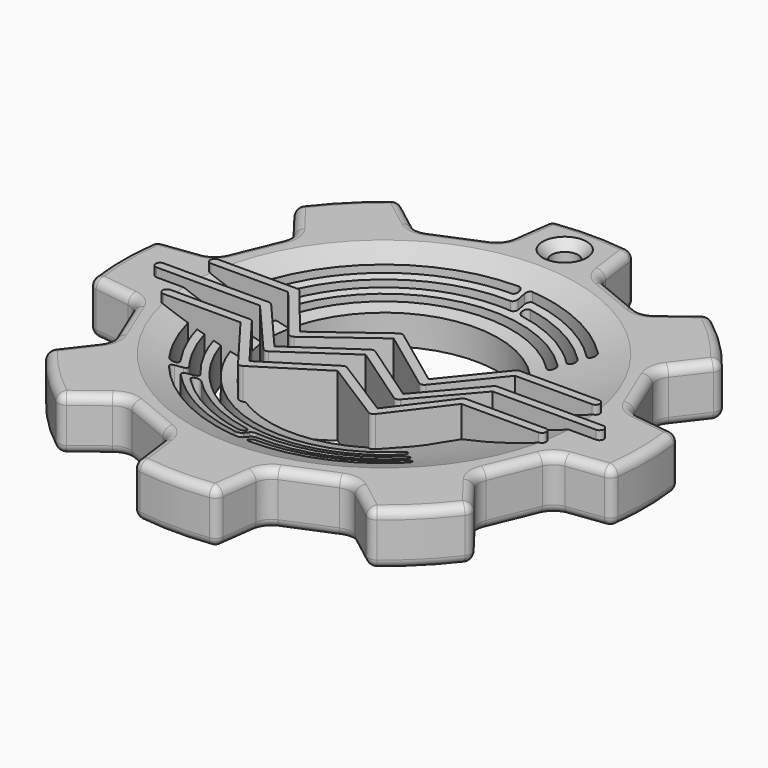
from build123d import *

# Parameters (mm, degrees)
F1_R          = 65
F3_DEPTH      = 15
F4_ANGLE      = 22.5
F5_DEPTH      = 37
F6_R          = 2.5
F7_R          = 10
F9_ANGLE_BACK = 42.021197958
F9_ANGLE      = 84.0423959161
F11_DEPTH     = 20
F12_DEPTH     = 15
F13_R         = 5
F14_R         = 7.5
F15_DEPTH     = 30.0010001
F16_SIZE      = 5


with BuildPart() as f3:
    # F1 (on Top) → F3 (new body, symmetric)
    with BuildSketch(Plane.XY):
        with BuildLine():
            Line((119.8787593446, 20), (145.8595214581, 35))
            ThreePointArc((145.8595214581, 35), (138.5819298767, 57.4025148548), (127.8869940652, 78.3895193822))
            Line((127.8869940652, 78.3895193822), (98.9092192765, 70.6249480291))
            Line((98.9092192765, 70.6249480291), (70.6249480291, 98.9092192765))
            Line((70.6249480291, 98.9092192765), (78.3895193822, 127.8869940652))
            ThreePointArc((78.3895193822, 127.8869940652), (57.4025148548, 138.5819298767), (35, 145.8595214581))
            Line((35, 145.8595214581), (20, 119.8787593446))
            Line((20, 119.8787593446), (-20, 119.8787593446))
            Line((-20, 119.8787593446), (-35, 145.8595214581))
            ThreePointArc((-35, 145.8595214581), (-57.4025148548, 138.5819298767), (-78.3895193822, 127.8869940652))
            Line((-78.3895193822, 127.8869940652), (-70.6249480291, 98.9092192765))
            Line((-70.6249480291, 98.9092192765), (-98.9092192765, 70.6249480291))
            Line((-98.9092192765, 70.6249480291), (-127.8869940652, 78.3895193822))
            ThreePointArc((-127.8869940652, 78.3895193822), (-138.5819298767, 57.4025148548), (-145.8595214581, 35))
            Line((-145.8595214581, 35), (-119.8787593446, 20))
            Line((-119.8787593446, 20), (-119.8787593446, -20))
            Line((-119.8787593446, -20), (-145.8595214581, -35))
            ThreePointArc((-145.8595214581, -35), (-138.5819298767, -57.4025148548), (-127.8869940652, -78.3895193822))
            Line((-127.8869940652, -78.3895193822), (-98.9092192765, -70.6249480291))
            Line((-98.9092192765, -70.6249480291), (-70.6249480291, -98.9092192765))
            Line((-70.6249480291, -98.9092192765), (-78.3895193822, -127.8869940652))
            ThreePointArc((-78.3895193822, -127.8869940652), (-57.4025148548, -138.5819298767), (-35, -145.8595214581))
            Line((-35, -145.8595214581), (-20, -119.8787593446))
            Line((-20, -119.8787593446), (20, -119.8787593446))
            Line((20, -119.8787593446), (35, -145.8595214581))
            ThreePointArc((35, -145.8595214581), (57.4025148548, -138.5819298767), (78.3895193822, -127.8869940652))
            Line((78.3895193822, -127.8869940652), (70.6249480291, -98.9092192765))
            Line((70.6249480291, -98.9092192765), (98.9092192765, -70.6249480291))
            Line((98.9092192765, -70.6249480291), (127.8869940652, -78.3895193822))
            ThreePointArc((127.8869940652, -78.3895193822), (138.5819298767, -57.4025148548), (145.8595214581, -35))
            Line((145.8595214581, -35), (119.8787593446, -20))
            Line((119.8787593446, -20), (119.8787593446, 20))
        make_face()
        Circle(F1_R, mode=Mode.SUBTRACT)
    extrude(amount=F3_DEPTH, both=True)


with BuildPart() as f3_1:
    # F4: moved
    add(f3.part.rotate(Axis((0, 0, -15), (0, 0, 1)), F4_ANGLE))

    # F0 (on Top) → F5 (cut, symmetric)
    with BuildSketch(Plane.XY):
        with BuildLine():
            ThreePointArc((51.265241636, 51.265241636), (54.800775542, 51.265241636), (54.800775542, 54.800775542))
            ThreePointArc((54.800775542, 54.800775542), (-77.5, 0), (54.800775542, -54.800775542))
            ThreePointArc((54.800775542, -54.800775542), (54.800775542, -51.265241636), (51.265241636, -51.265241636))
            ThreePointArc((51.265241636, -51.265241636), (-72.5, 0), (51.265241636, 51.265241636))
        make_face()
        with BuildLine():
            ThreePointArc((57.6292026667, 57.6292026667), (61.1647365726, 57.6292026667), (61.1647365726, 61.1647365726))
            ThreePointArc((61.1647365726, 61.1647365726), (39.9412550448, 76.7264370699), (15.0205673682, 85.1858706356))
            ThreePointArc((15.0205673682, 85.1858706356), (12.1244275415, 83.1579716972), (14.1523264799, 80.2618318705))
            ThreePointArc((14.1523264799, 80.2618318705), (37.6325119787, 72.291382904), (57.6292026667, 57.6292026667))
        make_face()
        with BuildLine():
            ThreePointArc((-62.7407641978, -55.9092703215), (-64.5656225789, -56.4846459589), (-66.2628443298, -55.6011282379))
            Line((-66.2628443298, -55.6011282379), (-69.3270221023, -58.1722786766))
            ThreePointArc((-69.3270221023, -58.1722786766), (-68.5168463916, -59.1243753502), (-67.6935962189, -60.0651898437))
            Line((-67.6935962189, -60.0651898437), (-62.7407641978, -55.9092703215))
        make_face()
        with BuildLine():
            ThreePointArc((-67.8421325563, -53.6627901829), (-67.0594922066, -54.6376656254), (-66.2628443298, -55.6011282379))
            ThreePointArc((-66.2628443298, -55.6011282379), (-64.5656225789, -56.4846459589), (-62.7407641978, -55.9092703215))
            ThreePointArc((-62.7407641978, -55.9092703215), (-61.8572464768, -54.2120485705), (-62.4326221142, -52.3871901895))
            ThreePointArc((-62.4326221142, -52.3871901895), (-64.1298438651, -51.5036724684), (-65.9547022462, -52.0790481059))
            Line((-65.9547022462, -52.0790481059), (-67.8421325563, -53.6627901829))
        make_face()
        with BuildLine():
            Line((-69.3270221023, -58.1722786766), (-66.2628443298, -55.6011282379))
            ThreePointArc((-66.2628443298, -55.6011282379), (-67.0594922066, -54.6376656254), (-67.8421325563, -53.6627901829))
            Line((-67.8421325563, -53.6627901829), (-72.8491022343, -57.8641365931))
            ThreePointArc((-72.8491022343, -57.8641365931), (-71.0242438532, -57.2887609556), (-69.3270221023, -58.1722786766))
        make_face()
        with BuildLine():
            ThreePointArc((-67.6935962189, -60.0651898437), (-68.5168463916, -59.1243753502), (-69.3270221023, -58.1722786766))
            ThreePointArc((-69.3270221023, -58.1722786766), (-71.0242438532, -57.2887609556), (-72.8491022343, -57.8641365931))
            ThreePointArc((-72.8491022343, -57.8641365931), (-73.7326199553, -59.561358344), (-73.1572443179, -61.3862167251))
            ThreePointArc((-73.1572443179, -61.3862167251), (-71.4600225669, -62.2697344461), (-69.6351641858, -61.6943588086))
            Line((-69.6351641858, -61.6943588086), (-67.6935962189, -60.0651898437))
        make_face()
        with BuildLine():
            ThreePointArc((5.0453356545, 86.3527335302), (-76.7264370699, 39.9412550448), (-67.8421325563, -53.6627901829))
            Line((-67.8421325563, -53.6627901829), (-65.9547022462, -52.0790481059))
            ThreePointArc((-65.9547022462, -52.0790481059), (-64.1298438651, -51.5036724684), (-62.4326221142, -52.3871901895))
            ThreePointArc((-62.4326221142, -52.3871901895), (-72.291382904, 37.6325119787), (7.1031930339, 81.1898678945))
            ThreePointArc((7.1031930339, 81.1898678945), (5.405971283, 82.0733856155), (4.8305956456, 83.8982439966))
            Line((4.8305956456, 83.8982439966), (5.0453356545, 86.3527335302))
        make_face()
        with BuildLine():
            ThreePointArc((-10.375071368, -89.9033252672), (-41.7882494978, -80.2744804026), (-67.6935962189, -60.0651898437))
            Line((-67.6935962189, -60.0651898437), (-69.6351641858, -61.6943588086))
            ThreePointArc((-69.6351641858, -61.6943588086), (-71.4600225669, -62.2697344461), (-73.1572443179, -61.3862167251))
            ThreePointArc((-73.1572443179, -61.3862167251), (-44.0969925639, -84.7095345685), (-8.3233734324, -95.1365936678))
            ThreePointArc((-8.3233734324, -95.1365936678), (-10.0205951833, -94.2530759467), (-10.5959708208, -92.4282175657))
            Line((-10.5959708208, -92.4282175657), (-10.375071368, -89.9033252672))
        make_face()
        with BuildLine():
            ThreePointArc((7.5389717477, 86.1708413849), (6.2928109289, 86.27079767), (5.0453356545, 86.3527335302))
            Line((5.0453356545, 86.3527335302), (4.8305956456, 83.8982439966))
            ThreePointArc((4.8305956456, 83.8982439966), (5.405971283, 82.0733856155), (7.1031930339, 81.1898678945))
            ThreePointArc((7.1031930339, 81.1898678945), (8.928051415, 81.7652435319), (9.811569136, 83.4624652828))
            ThreePointArc((9.811569136, 83.4624652828), (9.2361934986, 85.2873236639), (7.5389717477, 86.1708413849))
        make_face()
        with BuildLine():
            Line((5.6149973303, 92.8639962794), (5.0453356545, 86.3527335302))
            ThreePointArc((5.0453356545, 86.3527335302), (6.2928109289, 86.27079767), (7.5389717477, 86.1708413849))
            ThreePointArc((7.5389717477, 86.1708413849), (9.2361934986, 85.2873236639), (9.811569136, 83.4624652828))
            Line((9.811569136, 83.4624652828), (10.375071368, 89.9033252672))
            ThreePointArc((10.375071368, 89.9033252672), (9.1322043521, 90.0380633048), (7.8875947187, 90.1556201773))
            ThreePointArc((7.8875947187, 90.1556201773), (6.1903729677, 91.0391378983), (5.6149973303, 92.8639962794))
        make_face()
        with BuildLine():
            ThreePointArc((-7.8875947187, -90.1556201773), (-9.1322043521, -90.0380633048), (-10.375071368, -89.9033252672))
            Line((-10.375071368, -89.9033252672), (-10.5959708208, -92.4282175657))
            ThreePointArc((-10.5959708208, -92.4282175657), (-10.0205951833, -94.2530759467), (-8.3233734324, -95.1365936678))
            ThreePointArc((-8.3233734324, -95.1365936678), (-6.4985150513, -94.5612180303), (-5.6149973303, -92.8639962794))
            ThreePointArc((-5.6149973303, -92.8639962794), (-6.1903729677, -91.0391378983), (-7.8875947187, -90.1556201773))
        make_face()
        with BuildLine():
            Line((-9.811569136, -83.4624652828), (-10.375071368, -89.9033252672))
            ThreePointArc((-10.375071368, -89.9033252672), (-9.1322043521, -90.0380633048), (-7.8875947187, -90.1556201773))
            ThreePointArc((-7.8875947187, -90.1556201773), (-6.1903729677, -91.0391378983), (-5.6149973303, -92.8639962794))
            Line((-5.6149973303, -92.8639962794), (-5.0453356545, -86.3527335302))
            ThreePointArc((-5.0453356545, -86.3527335302), (-6.2928109289, -86.27079767), (-7.5389717477, -86.1708413849))
            ThreePointArc((-7.5389717477, -86.1708413849), (-9.2361934986, -85.2873236639), (-9.811569136, -83.4624652828))
        make_face()
        with BuildLine():
            ThreePointArc((8.3233734324, 95.1365936678), (6.4985150513, 94.5612180303), (5.6149973303, 92.8639962794))
            ThreePointArc((5.6149973303, 92.8639962794), (6.1903729677, 91.0391378983), (7.8875947187, 90.1556201773))
            ThreePointArc((7.8875947187, 90.1556201773), (9.1322043521, 90.0380633048), (10.375071368, 89.9033252672))
            Line((10.375071368, 89.9033252672), (10.5959708208, 92.4282175657))
            ThreePointArc((10.5959708208, 92.4282175657), (10.0205951833, 94.2530759467), (8.3233734324, 95.1365936678))
        make_face()
        with BuildLine():
            ThreePointArc((-7.1031930339, -81.1898678945), (-8.928051415, -81.7652435319), (-9.811569136, -83.4624652828))
            ThreePointArc((-9.811569136, -83.4624652828), (-9.2361934986, -85.2873236639), (-7.5389717477, -86.1708413849))
            ThreePointArc((-7.5389717477, -86.1708413849), (-6.2928109289, -86.27079767), (-5.0453356545, -86.3527335302))
            Line((-5.0453356545, -86.3527335302), (-4.8305956456, -83.8982439966))
            ThreePointArc((-4.8305956456, -83.8982439966), (-5.405971283, -82.0733856155), (-7.1031930339, -81.1898678945))
        make_face()
        with BuildLine():
            ThreePointArc((67.5286976033, 67.5286976033), (40.3600439962, 86.552393662), (8.3233734324, 95.1365936678))
            ThreePointArc((8.3233734324, 95.1365936678), (10.0205951833, 94.2530759467), (10.5959708208, 92.4282175657))
            Line((10.5959708208, 92.4282175657), (10.375071368, 89.9033252672))
            ThreePointArc((10.375071368, 89.9033252672), (39.3762963575, 81.4847058359), (63.9931636974, 63.9931636974))
            ThreePointArc((63.9931636974, 63.9931636974), (67.5286976033, 63.9931636974), (67.5286976033, 67.5286976033))
        make_face()
        with BuildLine():
            ThreePointArc((57.6292026667, -57.6292026667), (27.874641681, -76.5849485941), (-7.1031930339, -81.1898678945))
            ThreePointArc((-7.1031930339, -81.1898678945), (-5.405971283, -82.0733856155), (-4.8305956456, -83.8982439966))
            Line((-4.8305956456, -83.8982439966), (-5.0453356545, -86.3527335302))
            ThreePointArc((-5.0453356545, -86.3527335302), (30.7563910031, -80.8473525384), (61.1647365726, -61.1647365726))
            ThreePointArc((61.1647365726, -61.1647365726), (61.1647365726, -57.6292026667), (57.6292026667, -57.6292026667))
        make_face()
        with BuildLine():
            ThreePointArc((0, 90.5), (2.5, 93), (0, 95.5))
            ThreePointArc((0, 95.5), (-84.7095345685, 44.0969925639), (-78.2290202296, -54.7765496715))
            ThreePointArc((-78.2290202296, -54.7765496715), (-74.747199028, -55.3904886914), (-74.1332600082, -51.9086674898))
            ThreePointArc((-74.1332600082, -51.9086674898), (-80.2744804026, 41.7882494978), (0, 90.5))
        make_face()
        with BuildLine():
            ThreePointArc((0, -90.5), (-2.5, -93), (0, -95.5))
            ThreePointArc((0, -95.5), (36.5462677909, -88.2304953548), (67.5286976033, -67.5286976033))
            ThreePointArc((67.5286976033, -67.5286976033), (67.5286976033, -63.9931636974), (63.9931636974, -63.9931636974))
            ThreePointArc((63.9931636974, -63.9931636974), (34.632850629, -83.6110976923), (0, -90.5))
        make_face()
        with BuildLine():
            ThreePointArc((-57.6292026667, -57.6292026667), (-61.1647365726, -57.6292026667), (-61.1647365726, -61.1647365726))
            ThreePointArc((-61.1647365726, -61.1647365726), (-39.9412550448, -76.7264370699), (-15.0205673682, -85.1858706356))
            ThreePointArc((-15.0205673682, -85.1858706356), (-12.1244275415, -83.1579716972), (-14.1523264799, -80.2618318705))
            ThreePointArc((-14.1523264799, -80.2618318705), (-37.6325119787, -72.291382904), (-57.6292026667, -57.6292026667))
        make_face()
    extrude(amount=F5_DEPTH, both=True, mode=Mode.SUBTRACT)

    # F6
    f6_edges = [f3_1.edges().sort_by_distance(p)[0] for p in [
        (-67.842133, -53.66279, 0),
        (-10.375071, -89.903325, 0),
        (-5.045336, -86.352734, 0),
        (-67.693596, -60.06519, 0),
        (10.375071, 89.903325, 0),
        (5.045336, 86.352734, 0),
    ]]
    fillet(f6_edges, radius=F6_R)

    # F7
    f7_edges = [f3_1.edges().sort_by_distance(p)[0] for p in [
        (-118.407201, 27.398024, 0),
        (-103.099863, 64.353206, 0),
        (-64.353206, 103.099863, 0),
        (-27.398024, 118.407201, 0),
        (27.398024, 118.407201, 0),
        (64.353206, 103.099863, 0),
        (103.099863, 64.353206, 0),
        (118.407201, 27.398024, 0),
        (118.407201, -27.398024, 0),
        (103.099863, -64.353206, 0),
        (64.353206, -103.099863, 0),
        (27.398024, -118.407201, 0),
        (-27.398024, -118.407201, 0),
        (-64.353206, -103.099863, 0),
        (-103.099863, -64.353206, 0),
        (-118.407201, -27.398024, 0),
    ]]
    fillet(f7_edges, radius=F7_R)


with BuildPart() as f9:
    # F8 (on Front) → F9 (revolve)
    with BuildSketch(Plane.XZ, mode=Mode.PRIVATE) as f9_sk:
        with BuildLine():
            Line((0, 305), (-310, 305))
            ThreePointArc((-310, 305), (0, -5), (310, 305))
            Line((310, 305), (0, 305))
        make_face()
    revolve(f9_sk.sketch.rotate(Axis((0, 0, 305), (1, 0, 0)), -F9_ANGLE_BACK), axis=Axis((0, 0, 305), (1, 0, 0)), revolution_arc=F9_ANGLE)


with BuildPart() as f3_2:
    add(f3_1.part)

    # F10: cut F9
    add(f9.part, mode=Mode.SUBTRACT)

    # F2 (on Top) → F11 (join)
    with BuildSketch(Plane.XY):
        with BuildLine():
            ThreePointArc((-106.5142259969, -18.5), (-109.0142259969, -21), (-106.5142259969, -23.5))
            Line((-106.5142259969, -23.5), (-62.7586036079, -23.5))
            Line((-62.7586036079, -23.5), (-63.5088106899, -22.5071933859))
            ThreePointArc((-63.5088106899, -22.5071933859), (-63.7523036838, -19.8859944939), (-61.5142259969, -18.5))
            Line((-61.5142259969, -18.5), (-106.5142259969, -18.5))
        make_face()
        with BuildLine():
            Line((-63.5088106899, -22.5071933859), (-62.7586036079, -23.5))
            Line((-62.7586036079, -23.5), (-61.5142259969, -23.5))
            ThreePointArc((-61.5142259969, -23.5), (-59.2761483101, -22.1140055061), (-59.5196413039, -19.4928066141))
            ThreePointArc((-59.5196413039, -19.4928066141), (-60.4002204908, -18.7619223131), (-61.5142259969, -18.5))
            ThreePointArc((-61.5142259969, -18.5), (-63.7523036838, -19.8859944939), (-63.5088106899, -22.5071933859))
        make_face()
        with BuildLine():
            Line((-61.5142259969, -23.5), (-62.7586036079, -23.5))
            Line((-62.7586036079, -23.5), (-38.994584693, -54.9487502495))
            ThreePointArc((-38.994584693, -54.9487502495), (-39.459840378, -52.9952550434), (-38.3379651856, -51.3297213675))
            Line((-38.3379651856, -51.3297213675), (-36.3933006484, -50.0976682776))
            Line((-36.3933006484, -50.0976682776), (-59.5196413039, -19.4928066141))
            ThreePointArc((-59.5196413039, -19.4928066141), (-59.2761483101, -22.1140055061), (-61.5142259969, -23.5))
        make_face()
        with BuildLine():
            ThreePointArc((-38.3379651856, -51.3297213675), (-39.459840378, -52.9952550434), (-38.994584693, -54.9487502495))
            ThreePointArc((-38.994584693, -54.9487502495), (-37.4463018202, -55.9013972416), (-35.6620348144, -55.5533923596))
            ThreePointArc((-35.6620348144, -55.5533923596), (-34.540159622, -53.8878586837), (-35.005415307, -51.9343634776))
            Line((-35.005415307, -51.9343634776), (-36.3933006484, -50.0976682776))
            Line((-36.3933006484, -50.0976682776), (-38.3379651856, -51.3297213675))
        make_face()
        with BuildLine():
            ThreePointArc((-35.005415307, -51.9343634776), (-34.540159622, -53.8878586837), (-35.6620348144, -55.5533923596))
            Line((-35.6620348144, -55.5533923596), (0, -32.9595108198))
            Line((0, -32.9595108198), (-1.3379651856, -32.111835496))
            ThreePointArc((-1.3379651856, -32.111835496), (-2.5, -30), (-1.3379651856, -27.888164504))
            Line((-1.3379651856, -27.888164504), (-36.3933006484, -50.0976682776))
            Line((-36.3933006484, -50.0976682776), (-35.005415307, -51.9343634776))
        make_face()
        with BuildLine():
            Line((-1.3379651856, -32.111835496), (0, -32.9595108198))
            Line((0, -32.9595108198), (1.3379651856, -32.111835496))
            ThreePointArc((1.3379651856, -32.111835496), (2.5, -30), (1.3379651856, -27.888164504))
            ThreePointArc((1.3379651856, -27.888164504), (0, -27.5), (-1.3379651856, -27.888164504))
            ThreePointArc((-1.3379651856, -27.888164504), (-2.5, -30), (-1.3379651856, -32.111835496))
        make_face()
        with BuildLine():
            Line((1.3379651856, -32.111835496), (0, -32.9595108198))
            Line((0, -32.9595108198), (35.6620348144, -55.5533923596))
            ThreePointArc((35.6620348144, -55.5533923596), (34.540159622, -53.8878586837), (35.005415307, -51.9343634776))
            Line((35.005415307, -51.9343634776), (36.3933006484, -50.0976682776))
            Line((36.3933006484, -50.0976682776), (1.3379651856, -27.888164504))
            ThreePointArc((1.3379651856, -27.888164504), (2.5, -30), (1.3379651856, -32.111835496))
        make_face()
        with BuildLine():
            ThreePointArc((35.005415307, -51.9343634776), (34.540159622, -53.8878586837), (35.6620348144, -55.5533923596))
            ThreePointArc((35.6620348144, -55.5533923596), (37.4463018202, -55.9013972416), (38.994584693, -54.9487502495))
            ThreePointArc((38.994584693, -54.9487502495), (39.459840378, -52.9952550434), (38.3379651856, -51.3297213675))
            Line((38.3379651856, -51.3297213675), (36.3933006484, -50.0976682776))
            Line((36.3933006484, -50.0976682776), (35.005415307, -51.9343634776))
        make_face()
        with BuildLine():
            ThreePointArc((38.3379651856, -51.3297213675), (39.459840378, -52.9952550434), (38.994584693, -54.9487502495))
            Line((38.994584693, -54.9487502495), (62.7586036079, -23.5))
            Line((62.7586036079, -23.5), (61.5142259969, -23.5))
            ThreePointArc((61.5142259969, -23.5), (59.2761483101, -22.1140055061), (59.5196413039, -19.4928066141))
            Line((59.5196413039, -19.4928066141), (36.3933006484, -50.0976682776))
            Line((36.3933006484, -50.0976682776), (38.3379651856, -51.3297213675))
        make_face()
        with BuildLine():
            Line((61.5142259969, -23.5), (62.7586036079, -23.5))
            Line((62.7586036079, -23.5), (63.5088106899, -22.5071933859))
            ThreePointArc((63.5088106899, -22.5071933859), (63.7523036838, -19.8859944939), (61.5142259969, -18.5))
            ThreePointArc((61.5142259969, -18.5), (60.4002204908, -18.7619223131), (59.5196413039, -19.4928066141))
            ThreePointArc((59.5196413039, -19.4928066141), (59.2761483101, -22.1140055061), (61.5142259969, -23.5))
        make_face()
        with BuildLine():
            Line((63.5088106899, -22.5071933859), (62.7586036079, -23.5))
            Line((62.7586036079, -23.5), (106.5142259969, -23.5))
            ThreePointArc((106.5142259969, -23.5), (109.0142259969, -21), (106.5142259969, -18.5))
            Line((106.5142259969, -18.5), (61.5142259969, -18.5))
            ThreePointArc((61.5142259969, -18.5), (63.7523036838, -19.8859944939), (63.5088106899, -22.5071933859))
        make_face()
        with BuildLine():
            ThreePointArc((-124.930732323, -0.5), (-127.430732323, -3), (-124.930732323, -5.5))
            Line((-124.930732323, -5.5), (-66.0772491679, -5.5))
            Line((-66.0772491679, -5.5), (-66.825300226, -4.6311383942))
            ThreePointArc((-66.825300226, -4.6311383942), (-67.2031589979, -1.9578498154), (-64.930732323, -0.5))
            Line((-64.930732323, -0.5), (-124.930732323, -0.5))
        make_face()
        with BuildLine():
            Line((-66.825300226, -4.6311383942), (-66.0772491679, -5.5))
            Line((-66.0772491679, -5.5), (-64.930732323, -5.5))
            ThreePointArc((-64.930732323, -5.5), (-62.6583056481, -4.0421501846), (-63.03616442, -1.3688616058))
            ThreePointArc((-63.03616442, -1.3688616058), (-63.8885821384, -0.7275733251), (-64.930732323, -0.5))
            ThreePointArc((-64.930732323, -0.5), (-67.2031589979, -1.9578498154), (-66.825300226, -4.6311383942))
        make_face()
        with BuildLine():
            Line((-64.930732323, -5.5), (-66.0772491679, -5.5))
            Line((-66.0772491679, -5.5), (-38.894567903, -37.0726952577))
            ThreePointArc((-38.894567903, -37.0726952577), (-39.479289508, -35.1204283293), (-38.4164754282, -33.381557504))
            Line((-38.4164754282, -33.381557504), (-36.5686042305, -32.1109434459))
            Line((-36.5686042305, -32.1109434459), (-63.03616442, -1.3688616058))
            ThreePointArc((-63.03616442, -1.3688616058), (-62.6583056481, -4.0421501846), (-64.930732323, -5.5))
        make_face()
        with BuildLine():
            ThreePointArc((-38.4164754282, -33.381557504), (-39.479289508, -35.1204283293), (-38.894567903, -37.0726952577))
            ThreePointArc((-38.894567903, -37.0726952577), (-37.3211285343, -37.9208463716), (-35.5835245718, -37.5015562231))
            ThreePointArc((-35.5835245718, -37.5015562231), (-34.520710492, -35.7626853978), (-35.105432097, -33.8104184694))
            Line((-35.105432097, -33.8104184694), (-36.5686042305, -32.1109434459))
            Line((-36.5686042305, -32.1109434459), (-38.4164754282, -33.381557504))
        make_face()
        with BuildLine():
            ThreePointArc((-35.105432097, -33.8104184694), (-34.520710492, -35.7626853978), (-35.5835245718, -37.5015562231))
            Line((-35.5835245718, -37.5015562231), (0, -13.0339815258))
            Line((0, -13.0339815258), (-1.4164754282, -12.0599993595))
            ThreePointArc((-1.4164754282, -12.0599993595), (-2.5, -10), (-1.4164754282, -7.9400006405))
            Line((-1.4164754282, -7.9400006405), (-36.5686042305, -32.1109434459))
            Line((-36.5686042305, -32.1109434459), (-35.105432097, -33.8104184694))
        make_face()
        with BuildLine():
            Line((-1.4164754282, -12.0599993595), (0, -13.0339815258))
            Line((0, -13.0339815258), (1.4164754282, -12.0599993595))
            ThreePointArc((1.4164754282, -12.0599993595), (2.5, -10), (1.4164754282, -7.9400006405))
            ThreePointArc((1.4164754282, -7.9400006405), (0, -7.5), (-1.4164754282, -7.9400006405))
            ThreePointArc((-1.4164754282, -7.9400006405), (-2.5, -10), (-1.4164754282, -12.0599993595))
        make_face()
        with BuildLine():
            Line((1.4164754282, -12.0599993595), (0, -13.0339815258))
            Line((0, -13.0339815258), (35.5835245718, -37.5015562231))
            ThreePointArc((35.5835245718, -37.5015562231), (34.520710492, -35.7626853978), (35.105432097, -33.8104184694))
            Line((35.105432097, -33.8104184694), (36.5686042305, -32.1109434459))
            Line((36.5686042305, -32.1109434459), (1.4164754282, -7.9400006405))
            ThreePointArc((1.4164754282, -7.9400006405), (2.5, -10), (1.4164754282, -12.0599993595))
        make_face()
        with BuildLine():
            ThreePointArc((35.105432097, -33.8104184694), (34.520710492, -35.7626853978), (35.5835245718, -37.5015562231))
            ThreePointArc((35.5835245718, -37.5015562231), (37.3211285343, -37.9208463716), (38.894567903, -37.0726952577))
            ThreePointArc((38.894567903, -37.0726952577), (39.479289508, -35.1204283293), (38.4164754282, -33.381557504))
            Line((38.4164754282, -33.381557504), (36.5686042305, -32.1109434459))
            Line((36.5686042305, -32.1109434459), (35.105432097, -33.8104184694))
        make_face()
        with BuildLine():
            ThreePointArc((38.4164754282, -33.381557504), (39.479289508, -35.1204283293), (38.894567903, -37.0726952577))
            Line((38.894567903, -37.0726952577), (66.0772491679, -5.5))
            Line((66.0772491679, -5.5), (64.930732323, -5.5))
            ThreePointArc((64.930732323, -5.5), (62.6583056481, -4.0421501846), (63.03616442, -1.3688616058))
            Line((63.03616442, -1.3688616058), (36.5686042305, -32.1109434459))
            Line((36.5686042305, -32.1109434459), (38.4164754282, -33.381557504))
        make_face()
        with BuildLine():
            Line((64.930732323, -5.5), (66.0772491679, -5.5))
            Line((66.0772491679, -5.5), (66.825300226, -4.6311383942))
            ThreePointArc((66.825300226, -4.6311383942), (67.2031589979, -1.9578498154), (64.930732323, -0.5))
            ThreePointArc((64.930732323, -0.5), (63.8885821384, -0.7275733251), (63.03616442, -1.3688616058))
            ThreePointArc((63.03616442, -1.3688616058), (62.6583056481, -4.0421501846), (64.930732323, -5.5))
        make_face()
        with BuildLine():
            Line((66.825300226, -4.6311383942), (66.0772491679, -5.5))
            Line((66.0772491679, -5.5), (124.930732323, -5.5))
            ThreePointArc((124.930732323, -5.5), (127.430732323, -3), (124.930732323, -0.5))
            Line((124.930732323, -0.5), (64.930732323, -0.5))
            ThreePointArc((64.930732323, -0.5), (67.2031589979, -1.9578498154), (66.825300226, -4.6311383942))
        make_face()
        with BuildLine():
            ThreePointArc((-108.2455532034, 17.5), (-110.7455532034, 15), (-108.2455532034, 12.5))
            Line((-108.2455532034, 12.5), (-64.4387094171, 12.5))
            Line((-64.4387094171, 12.5), (-65.1891533907, 13.4276074562))
            ThreePointArc((-65.1891533907, 13.4276074562), (-65.5017647803, 16.076805145), (-63.2455532034, 17.5))
            Line((-63.2455532034, 17.5), (-108.2455532034, 17.5))
        make_face()
        with BuildLine():
            Line((-65.1891533907, 13.4276074562), (-64.4387094171, 12.5))
            Line((-64.4387094171, 12.5), (-63.2455532034, 12.5))
            ThreePointArc((-63.2455532034, 12.5), (-60.9893416265, 13.923194855), (-61.3019530161, 16.5723925438))
            ThreePointArc((-61.3019530161, 16.5723925438), (-62.1687480584, 17.2562115769), (-63.2455532034, 17.5))
            ThreePointArc((-63.2455532034, 17.5), (-65.5017647803, 16.076805145), (-65.1891533907, 13.4276074562))
        make_face()
        with BuildLine():
            Line((-63.2455532034, 12.5), (-64.4387094171, 12.5))
            Line((-64.4387094171, 12.5), (-38.9436001873, -19.0139494074))
            ThreePointArc((-38.9436001873, -19.0139494074), (-39.4801119208, -17.1268429298), (-38.4892652999, -15.4335506717))
            Line((-38.4892652999, -15.4335506717), (-36.56400064, -14.0056517625))
            Line((-36.56400064, -14.0056517625), (-61.3019530161, 16.5723925438))
            ThreePointArc((-61.3019530161, 16.5723925438), (-60.9893416265, 13.923194855), (-63.2455532034, 12.5))
        make_face()
        with BuildLine():
            ThreePointArc((-38.4892652999, -15.4335506717), (-39.4801119208, -17.1268429298), (-38.9436001873, -19.0139494074))
            ThreePointArc((-38.9436001873, -19.0139494074), (-37.3147139337, -19.9216687844), (-35.5107347001, -19.4495630554))
            ThreePointArc((-35.5107347001, -19.4495630554), (-34.5198880792, -17.7562707973), (-35.0563998127, -15.8691643197))
            Line((-35.0563998127, -15.8691643197), (-36.56400064, -14.0056517625))
            Line((-36.56400064, -14.0056517625), (-38.4892652999, -15.4335506717))
        make_face()
        with BuildLine():
            ThreePointArc((-35.0563998127, -15.8691643197), (-34.5198880792, -17.7562707973), (-35.5107347001, -19.4495630554))
            Line((-35.5107347001, -19.4495630554), (0, 6.887459797))
            Line((0, 6.887459797), (-1.4892652999, 7.9919938081))
            ThreePointArc((-1.4892652999, 7.9919938081), (-2.5, 10), (-1.4892652999, 12.0080061919))
            Line((-1.4892652999, 12.0080061919), (-36.56400064, -14.0056517625))
            Line((-36.56400064, -14.0056517625), (-35.0563998127, -15.8691643197))
        make_face()
        with BuildLine():
            Line((-1.4892652999, 7.9919938081), (0, 6.887459797))
            Line((0, 6.887459797), (1.4892652999, 7.9919938081))
            ThreePointArc((1.4892652999, 7.9919938081), (2.5, 10), (1.4892652999, 12.0080061919))
            ThreePointArc((1.4892652999, 12.0080061919), (0, 12.5), (-1.4892652999, 12.0080061919))
            ThreePointArc((-1.4892652999, 12.0080061919), (-2.5, 10), (-1.4892652999, 7.9919938081))
        make_face()
        with BuildLine():
            Line((1.4892652999, 7.9919938081), (0, 6.887459797))
            Line((0, 6.887459797), (35.5107347001, -19.4495630554))
            ThreePointArc((35.5107347001, -19.4495630554), (34.5198880792, -17.7562707973), (35.0563998127, -15.8691643197))
            Line((35.0563998127, -15.8691643197), (36.56400064, -14.0056517625))
            Line((36.56400064, -14.0056517625), (1.4892652999, 12.0080061919))
            ThreePointArc((1.4892652999, 12.0080061919), (2.5, 10), (1.4892652999, 7.9919938081))
        make_face()
        with BuildLine():
            ThreePointArc((35.0563998127, -15.8691643197), (34.5198880792, -17.7562707973), (35.5107347001, -19.4495630554))
            ThreePointArc((35.5107347001, -19.4495630554), (37.3147139337, -19.9216687844), (38.9436001873, -19.0139494074))
            ThreePointArc((38.9436001873, -19.0139494074), (39.4801119208, -17.1268429298), (38.4892652999, -15.4335506717))
            Line((38.4892652999, -15.4335506717), (36.56400064, -14.0056517625))
            Line((36.56400064, -14.0056517625), (35.0563998127, -15.8691643197))
        make_face()
        with BuildLine():
            ThreePointArc((38.4892652999, -15.4335506717), (39.4801119208, -17.1268429298), (38.9436001873, -19.0139494074))
            Line((38.9436001873, -19.0139494074), (64.4387094171, 12.5))
            Line((64.4387094171, 12.5), (63.2455532034, 12.5))
            ThreePointArc((63.2455532034, 12.5), (60.9893416265, 13.923194855), (61.3019530161, 16.5723925438))
            Line((61.3019530161, 16.5723925438), (36.56400064, -14.0056517625))
            Line((36.56400064, -14.0056517625), (38.4892652999, -15.4335506717))
        make_face()
        with BuildLine():
            Line((63.2455532034, 12.5), (64.4387094171, 12.5))
            Line((64.4387094171, 12.5), (65.1891533907, 13.4276074562))
            ThreePointArc((65.1891533907, 13.4276074562), (65.5017647803, 16.076805145), (63.2455532034, 17.5))
            ThreePointArc((63.2455532034, 17.5), (62.1687480584, 17.2562115769), (61.3019530161, 16.5723925438))
            ThreePointArc((61.3019530161, 16.5723925438), (60.9893416265, 13.923194855), (63.2455532034, 12.5))
        make_face()
        with BuildLine():
            Line((65.1891533907, 13.4276074562), (64.4387094171, 12.5))
            Line((64.4387094171, 12.5), (108.2455532034, 12.5))
            ThreePointArc((108.2455532034, 12.5), (110.7455532034, 15), (108.2455532034, 17.5))
            Line((108.2455532034, 17.5), (63.2455532034, 17.5))
            ThreePointArc((63.2455532034, 17.5), (65.5017647803, 16.076805145), (65.1891533907, 13.4276074562))
        make_face()
    extrude(amount=F11_DEPTH)

    # F2 (on Top) → F12 (join)
    with BuildSketch(Plane.XY):
        with BuildLine():
            ThreePointArc((-106.5142259969, -18.5), (-109.0142259969, -21), (-106.5142259969, -23.5))
            Line((-106.5142259969, -23.5), (-62.7586036079, -23.5))
            Line((-62.7586036079, -23.5), (-63.5088106899, -22.5071933859))
            ThreePointArc((-63.5088106899, -22.5071933859), (-63.7523036838, -19.8859944939), (-61.5142259969, -18.5))
            Line((-61.5142259969, -18.5), (-106.5142259969, -18.5))
        make_face()
        with BuildLine():
            Line((-63.5088106899, -22.5071933859), (-62.7586036079, -23.5))
            Line((-62.7586036079, -23.5), (-61.5142259969, -23.5))
            ThreePointArc((-61.5142259969, -23.5), (-59.2761483101, -22.1140055061), (-59.5196413039, -19.4928066141))
            ThreePointArc((-59.5196413039, -19.4928066141), (-60.4002204908, -18.7619223131), (-61.5142259969, -18.5))
            ThreePointArc((-61.5142259969, -18.5), (-63.7523036838, -19.8859944939), (-63.5088106899, -22.5071933859))
        make_face()
        with BuildLine():
            Line((-61.5142259969, -23.5), (-62.7586036079, -23.5))
            Line((-62.7586036079, -23.5), (-38.994584693, -54.9487502495))
            ThreePointArc((-38.994584693, -54.9487502495), (-39.459840378, -52.9952550434), (-38.3379651856, -51.3297213675))
            Line((-38.3379651856, -51.3297213675), (-36.3933006484, -50.0976682776))
            Line((-36.3933006484, -50.0976682776), (-59.5196413039, -19.4928066141))
            ThreePointArc((-59.5196413039, -19.4928066141), (-59.2761483101, -22.1140055061), (-61.5142259969, -23.5))
        make_face()
        with BuildLine():
            ThreePointArc((-38.3379651856, -51.3297213675), (-39.459840378, -52.9952550434), (-38.994584693, -54.9487502495))
            ThreePointArc((-38.994584693, -54.9487502495), (-37.4463018202, -55.9013972416), (-35.6620348144, -55.5533923596))
            ThreePointArc((-35.6620348144, -55.5533923596), (-34.540159622, -53.8878586837), (-35.005415307, -51.9343634776))
            Line((-35.005415307, -51.9343634776), (-36.3933006484, -50.0976682776))
            Line((-36.3933006484, -50.0976682776), (-38.3379651856, -51.3297213675))
        make_face()
        with BuildLine():
            ThreePointArc((-35.005415307, -51.9343634776), (-34.540159622, -53.8878586837), (-35.6620348144, -55.5533923596))
            Line((-35.6620348144, -55.5533923596), (0, -32.9595108198))
            Line((0, -32.9595108198), (-1.3379651856, -32.111835496))
            ThreePointArc((-1.3379651856, -32.111835496), (-2.5, -30), (-1.3379651856, -27.888164504))
            Line((-1.3379651856, -27.888164504), (-36.3933006484, -50.0976682776))
            Line((-36.3933006484, -50.0976682776), (-35.005415307, -51.9343634776))
        make_face()
        with BuildLine():
            Line((-1.3379651856, -32.111835496), (0, -32.9595108198))
            Line((0, -32.9595108198), (1.3379651856, -32.111835496))
            ThreePointArc((1.3379651856, -32.111835496), (2.5, -30), (1.3379651856, -27.888164504))
            ThreePointArc((1.3379651856, -27.888164504), (0, -27.5), (-1.3379651856, -27.888164504))
            ThreePointArc((-1.3379651856, -27.888164504), (-2.5, -30), (-1.3379651856, -32.111835496))
        make_face()
        with BuildLine():
            Line((1.3379651856, -32.111835496), (0, -32.9595108198))
            Line((0, -32.9595108198), (35.6620348144, -55.5533923596))
            ThreePointArc((35.6620348144, -55.5533923596), (34.540159622, -53.8878586837), (35.005415307, -51.9343634776))
            Line((35.005415307, -51.9343634776), (36.3933006484, -50.0976682776))
            Line((36.3933006484, -50.0976682776), (1.3379651856, -27.888164504))
            ThreePointArc((1.3379651856, -27.888164504), (2.5, -30), (1.3379651856, -32.111835496))
        make_face()
        with BuildLine():
            ThreePointArc((35.005415307, -51.9343634776), (34.540159622, -53.8878586837), (35.6620348144, -55.5533923596))
            ThreePointArc((35.6620348144, -55.5533923596), (37.4463018202, -55.9013972416), (38.994584693, -54.9487502495))
            ThreePointArc((38.994584693, -54.9487502495), (39.459840378, -52.9952550434), (38.3379651856, -51.3297213675))
            Line((38.3379651856, -51.3297213675), (36.3933006484, -50.0976682776))
            Line((36.3933006484, -50.0976682776), (35.005415307, -51.9343634776))
        make_face()
        with BuildLine():
            ThreePointArc((38.3379651856, -51.3297213675), (39.459840378, -52.9952550434), (38.994584693, -54.9487502495))
            Line((38.994584693, -54.9487502495), (62.7586036079, -23.5))
            Line((62.7586036079, -23.5), (61.5142259969, -23.5))
            ThreePointArc((61.5142259969, -23.5), (59.2761483101, -22.1140055061), (59.5196413039, -19.4928066141))
            Line((59.5196413039, -19.4928066141), (36.3933006484, -50.0976682776))
            Line((36.3933006484, -50.0976682776), (38.3379651856, -51.3297213675))
        make_face()
        with BuildLine():
            Line((61.5142259969, -23.5), (62.7586036079, -23.5))
            Line((62.7586036079, -23.5), (63.5088106899, -22.5071933859))
            ThreePointArc((63.5088106899, -22.5071933859), (63.7523036838, -19.8859944939), (61.5142259969, -18.5))
            ThreePointArc((61.5142259969, -18.5), (60.4002204908, -18.7619223131), (59.5196413039, -19.4928066141))
            ThreePointArc((59.5196413039, -19.4928066141), (59.2761483101, -22.1140055061), (61.5142259969, -23.5))
        make_face()
        with BuildLine():
            Line((63.5088106899, -22.5071933859), (62.7586036079, -23.5))
            Line((62.7586036079, -23.5), (106.5142259969, -23.5))
            ThreePointArc((106.5142259969, -23.5), (109.0142259969, -21), (106.5142259969, -18.5))
            Line((106.5142259969, -18.5), (61.5142259969, -18.5))
            ThreePointArc((61.5142259969, -18.5), (63.7523036838, -19.8859944939), (63.5088106899, -22.5071933859))
        make_face()
        with BuildLine():
            ThreePointArc((-124.930732323, -0.5), (-127.430732323, -3), (-124.930732323, -5.5))
            Line((-124.930732323, -5.5), (-66.0772491679, -5.5))
            Line((-66.0772491679, -5.5), (-66.825300226, -4.6311383942))
            ThreePointArc((-66.825300226, -4.6311383942), (-67.2031589979, -1.9578498154), (-64.930732323, -0.5))
            Line((-64.930732323, -0.5), (-124.930732323, -0.5))
        make_face()
        with BuildLine():
            Line((-66.825300226, -4.6311383942), (-66.0772491679, -5.5))
            Line((-66.0772491679, -5.5), (-64.930732323, -5.5))
            ThreePointArc((-64.930732323, -5.5), (-62.6583056481, -4.0421501846), (-63.03616442, -1.3688616058))
            ThreePointArc((-63.03616442, -1.3688616058), (-63.8885821384, -0.7275733251), (-64.930732323, -0.5))
            ThreePointArc((-64.930732323, -0.5), (-67.2031589979, -1.9578498154), (-66.825300226, -4.6311383942))
        make_face()
        with BuildLine():
            Line((-64.930732323, -5.5), (-66.0772491679, -5.5))
            Line((-66.0772491679, -5.5), (-38.894567903, -37.0726952577))
            ThreePointArc((-38.894567903, -37.0726952577), (-39.479289508, -35.1204283293), (-38.4164754282, -33.381557504))
            Line((-38.4164754282, -33.381557504), (-36.5686042305, -32.1109434459))
            Line((-36.5686042305, -32.1109434459), (-63.03616442, -1.3688616058))
            ThreePointArc((-63.03616442, -1.3688616058), (-62.6583056481, -4.0421501846), (-64.930732323, -5.5))
        make_face()
        with BuildLine():
            ThreePointArc((-38.4164754282, -33.381557504), (-39.479289508, -35.1204283293), (-38.894567903, -37.0726952577))
            ThreePointArc((-38.894567903, -37.0726952577), (-37.3211285343, -37.9208463716), (-35.5835245718, -37.5015562231))
            ThreePointArc((-35.5835245718, -37.5015562231), (-34.520710492, -35.7626853978), (-35.105432097, -33.8104184694))
            Line((-35.105432097, -33.8104184694), (-36.5686042305, -32.1109434459))
            Line((-36.5686042305, -32.1109434459), (-38.4164754282, -33.381557504))
        make_face()
        with BuildLine():
            ThreePointArc((-35.105432097, -33.8104184694), (-34.520710492, -35.7626853978), (-35.5835245718, -37.5015562231))
            Line((-35.5835245718, -37.5015562231), (0, -13.0339815258))
            Line((0, -13.0339815258), (-1.4164754282, -12.0599993595))
            ThreePointArc((-1.4164754282, -12.0599993595), (-2.5, -10), (-1.4164754282, -7.9400006405))
            Line((-1.4164754282, -7.9400006405), (-36.5686042305, -32.1109434459))
            Line((-36.5686042305, -32.1109434459), (-35.105432097, -33.8104184694))
        make_face()
        with BuildLine():
            Line((-1.4164754282, -12.0599993595), (0, -13.0339815258))
            Line((0, -13.0339815258), (1.4164754282, -12.0599993595))
            ThreePointArc((1.4164754282, -12.0599993595), (2.5, -10), (1.4164754282, -7.9400006405))
            ThreePointArc((1.4164754282, -7.9400006405), (0, -7.5), (-1.4164754282, -7.9400006405))
            ThreePointArc((-1.4164754282, -7.9400006405), (-2.5, -10), (-1.4164754282, -12.0599993595))
        make_face()
        with BuildLine():
            Line((1.4164754282, -12.0599993595), (0, -13.0339815258))
            Line((0, -13.0339815258), (35.5835245718, -37.5015562231))
            ThreePointArc((35.5835245718, -37.5015562231), (34.520710492, -35.7626853978), (35.105432097, -33.8104184694))
            Line((35.105432097, -33.8104184694), (36.5686042305, -32.1109434459))
            Line((36.5686042305, -32.1109434459), (1.4164754282, -7.9400006405))
            ThreePointArc((1.4164754282, -7.9400006405), (2.5, -10), (1.4164754282, -12.0599993595))
        make_face()
        with BuildLine():
            ThreePointArc((35.105432097, -33.8104184694), (34.520710492, -35.7626853978), (35.5835245718, -37.5015562231))
            ThreePointArc((35.5835245718, -37.5015562231), (37.3211285343, -37.9208463716), (38.894567903, -37.0726952577))
            ThreePointArc((38.894567903, -37.0726952577), (39.479289508, -35.1204283293), (38.4164754282, -33.381557504))
            Line((38.4164754282, -33.381557504), (36.5686042305, -32.1109434459))
            Line((36.5686042305, -32.1109434459), (35.105432097, -33.8104184694))
        make_face()
        with BuildLine():
            ThreePointArc((38.4164754282, -33.381557504), (39.479289508, -35.1204283293), (38.894567903, -37.0726952577))
            Line((38.894567903, -37.0726952577), (66.0772491679, -5.5))
            Line((66.0772491679, -5.5), (64.930732323, -5.5))
            ThreePointArc((64.930732323, -5.5), (62.6583056481, -4.0421501846), (63.03616442, -1.3688616058))
            Line((63.03616442, -1.3688616058), (36.5686042305, -32.1109434459))
            Line((36.5686042305, -32.1109434459), (38.4164754282, -33.381557504))
        make_face()
        with BuildLine():
            Line((64.930732323, -5.5), (66.0772491679, -5.5))
            Line((66.0772491679, -5.5), (66.825300226, -4.6311383942))
            ThreePointArc((66.825300226, -4.6311383942), (67.2031589979, -1.9578498154), (64.930732323, -0.5))
            ThreePointArc((64.930732323, -0.5), (63.8885821384, -0.7275733251), (63.03616442, -1.3688616058))
            ThreePointArc((63.03616442, -1.3688616058), (62.6583056481, -4.0421501846), (64.930732323, -5.5))
        make_face()
        with BuildLine():
            Line((66.825300226, -4.6311383942), (66.0772491679, -5.5))
            Line((66.0772491679, -5.5), (124.930732323, -5.5))
            ThreePointArc((124.930732323, -5.5), (127.430732323, -3), (124.930732323, -0.5))
            Line((124.930732323, -0.5), (64.930732323, -0.5))
            ThreePointArc((64.930732323, -0.5), (67.2031589979, -1.9578498154), (66.825300226, -4.6311383942))
        make_face()
        with BuildLine():
            ThreePointArc((-108.2455532034, 17.5), (-110.7455532034, 15), (-108.2455532034, 12.5))
            Line((-108.2455532034, 12.5), (-64.4387094171, 12.5))
            Line((-64.4387094171, 12.5), (-65.1891533907, 13.4276074562))
            ThreePointArc((-65.1891533907, 13.4276074562), (-65.5017647803, 16.076805145), (-63.2455532034, 17.5))
            Line((-63.2455532034, 17.5), (-108.2455532034, 17.5))
        make_face()
        with BuildLine():
            Line((-65.1891533907, 13.4276074562), (-64.4387094171, 12.5))
            Line((-64.4387094171, 12.5), (-63.2455532034, 12.5))
            ThreePointArc((-63.2455532034, 12.5), (-60.9893416265, 13.923194855), (-61.3019530161, 16.5723925438))
            ThreePointArc((-61.3019530161, 16.5723925438), (-62.1687480584, 17.2562115769), (-63.2455532034, 17.5))
            ThreePointArc((-63.2455532034, 17.5), (-65.5017647803, 16.076805145), (-65.1891533907, 13.4276074562))
        make_face()
        with BuildLine():
            Line((-63.2455532034, 12.5), (-64.4387094171, 12.5))
            Line((-64.4387094171, 12.5), (-38.9436001873, -19.0139494074))
            ThreePointArc((-38.9436001873, -19.0139494074), (-39.4801119208, -17.1268429298), (-38.4892652999, -15.4335506717))
            Line((-38.4892652999, -15.4335506717), (-36.56400064, -14.0056517625))
            Line((-36.56400064, -14.0056517625), (-61.3019530161, 16.5723925438))
            ThreePointArc((-61.3019530161, 16.5723925438), (-60.9893416265, 13.923194855), (-63.2455532034, 12.5))
        make_face()
        with BuildLine():
            ThreePointArc((-38.4892652999, -15.4335506717), (-39.4801119208, -17.1268429298), (-38.9436001873, -19.0139494074))
            ThreePointArc((-38.9436001873, -19.0139494074), (-37.3147139337, -19.9216687844), (-35.5107347001, -19.4495630554))
            ThreePointArc((-35.5107347001, -19.4495630554), (-34.5198880792, -17.7562707973), (-35.0563998127, -15.8691643197))
            Line((-35.0563998127, -15.8691643197), (-36.56400064, -14.0056517625))
            Line((-36.56400064, -14.0056517625), (-38.4892652999, -15.4335506717))
        make_face()
        with BuildLine():
            ThreePointArc((-35.0563998127, -15.8691643197), (-34.5198880792, -17.7562707973), (-35.5107347001, -19.4495630554))
            Line((-35.5107347001, -19.4495630554), (0, 6.887459797))
            Line((0, 6.887459797), (-1.4892652999, 7.9919938081))
            ThreePointArc((-1.4892652999, 7.9919938081), (-2.5, 10), (-1.4892652999, 12.0080061919))
            Line((-1.4892652999, 12.0080061919), (-36.56400064, -14.0056517625))
            Line((-36.56400064, -14.0056517625), (-35.0563998127, -15.8691643197))
        make_face()
        with BuildLine():
            Line((-1.4892652999, 7.9919938081), (0, 6.887459797))
            Line((0, 6.887459797), (1.4892652999, 7.9919938081))
            ThreePointArc((1.4892652999, 7.9919938081), (2.5, 10), (1.4892652999, 12.0080061919))
            ThreePointArc((1.4892652999, 12.0080061919), (0, 12.5), (-1.4892652999, 12.0080061919))
            ThreePointArc((-1.4892652999, 12.0080061919), (-2.5, 10), (-1.4892652999, 7.9919938081))
        make_face()
        with BuildLine():
            Line((1.4892652999, 7.9919938081), (0, 6.887459797))
            Line((0, 6.887459797), (35.5107347001, -19.4495630554))
            ThreePointArc((35.5107347001, -19.4495630554), (34.5198880792, -17.7562707973), (35.0563998127, -15.8691643197))
            Line((35.0563998127, -15.8691643197), (36.56400064, -14.0056517625))
            Line((36.56400064, -14.0056517625), (1.4892652999, 12.0080061919))
            ThreePointArc((1.4892652999, 12.0080061919), (2.5, 10), (1.4892652999, 7.9919938081))
        make_face()
        with BuildLine():
            ThreePointArc((35.0563998127, -15.8691643197), (34.5198880792, -17.7562707973), (35.5107347001, -19.4495630554))
            ThreePointArc((35.5107347001, -19.4495630554), (37.3147139337, -19.9216687844), (38.9436001873, -19.0139494074))
            ThreePointArc((38.9436001873, -19.0139494074), (39.4801119208, -17.1268429298), (38.4892652999, -15.4335506717))
            Line((38.4892652999, -15.4335506717), (36.56400064, -14.0056517625))
            Line((36.56400064, -14.0056517625), (35.0563998127, -15.8691643197))
        make_face()
        with BuildLine():
            ThreePointArc((38.4892652999, -15.4335506717), (39.4801119208, -17.1268429298), (38.9436001873, -19.0139494074))
            Line((38.9436001873, -19.0139494074), (64.4387094171, 12.5))
            Line((64.4387094171, 12.5), (63.2455532034, 12.5))
            ThreePointArc((63.2455532034, 12.5), (60.9893416265, 13.923194855), (61.3019530161, 16.5723925438))
            Line((61.3019530161, 16.5723925438), (36.56400064, -14.0056517625))
            Line((36.56400064, -14.0056517625), (38.4892652999, -15.4335506717))
        make_face()
        with BuildLine():
            Line((63.2455532034, 12.5), (64.4387094171, 12.5))
            Line((64.4387094171, 12.5), (65.1891533907, 13.4276074562))
            ThreePointArc((65.1891533907, 13.4276074562), (65.5017647803, 16.076805145), (63.2455532034, 17.5))
            ThreePointArc((63.2455532034, 17.5), (62.1687480584, 17.2562115769), (61.3019530161, 16.5723925438))
            ThreePointArc((61.3019530161, 16.5723925438), (60.9893416265, 13.923194855), (63.2455532034, 12.5))
        make_face()
        with BuildLine():
            Line((65.1891533907, 13.4276074562), (64.4387094171, 12.5))
            Line((64.4387094171, 12.5), (108.2455532034, 12.5))
            ThreePointArc((108.2455532034, 12.5), (110.7455532034, 15), (108.2455532034, 17.5))
            Line((108.2455532034, 17.5), (63.2455532034, 17.5))
            ThreePointArc((63.2455532034, 17.5), (65.5017647803, 16.076805145), (65.1891533907, 13.4276074562))
        make_face()
    extrude(amount=-F12_DEPTH)

    # F13
    f13_edges = [f3_2.edges().sort_by_distance(p)[0] for p in [
        (-110.753532, -45.875615, -15),
        (-116.197777, -32.732045, 0),
        (-105.309287, -59.019185, 0),
        (-110.753532, -45.875615, 15),
        (-136.140928, -25.063335, -15),
        (-124.13131, -26.644431, 0),
        (-148.150547, -23.482239, 0),
        (-136.140928, -25.063335, 15),
        (-148.150547, 23.482239, 0),
        (-150, 0, -15),
        (-150, 0, 15),
        (-113.988628, -78.54372, -15),
        (-106.614549, -68.933633, 0),
        (-121.362706, -88.153806, 0),
        (-113.988628, -78.54372, 15),
        (-106.066017, -106.066017, -15),
        (-88.153806, -121.362706, 0),
        (-106.066017, -106.066017, 15),
        (-78.54372, -113.988628, -15),
        (-68.933633, -106.614549, 0),
        (-78.54372, -113.988628, 15),
        (-45.875615, -110.753532, -15),
        (-59.019185, -105.309287, 0),
        (-32.732045, -116.197777, 0),
        (-45.875615, -110.753532, 15),
        (-23.482239, -148.150547, 0),
        (0, -150, -15),
        (23.482239, -148.150547, 0),
        (0, -150, 15),
        (-25.063335, -136.140928, -15),
        (-26.644431, -124.13131, 0),
        (-25.063335, -136.140928, 15),
        (25.063335, -136.140928, -15),
        (26.644431, -124.13131, 0),
        (25.063335, -136.140928, 15),
        (45.875615, -110.753532, -15),
        (32.732045, -116.197777, 0),
        (59.019185, -105.309287, 0),
        (45.875615, -110.753532, 15),
        (78.54372, -113.988628, -15),
        (68.933633, -106.614549, 0),
        (88.153806, -121.362706, 0),
        (78.54372, -113.988628, 15),
        (106.066017, -106.066017, -15),
        (121.362706, -88.153806, 0),
        (106.066017, -106.066017, 15),
        (113.988628, -78.54372, -15),
        (106.614549, -68.933633, 0),
        (113.988628, -78.54372, 15),
        (110.753532, -45.875615, -15),
        (105.309287, -59.019185, 0),
        (116.197777, -32.732045, 0),
        (110.753532, -45.875615, 15),
        (136.140928, -25.063335, -15),
        (124.13131, -26.644431, 0),
        (148.150547, -23.482239, 0),
        (136.140928, -25.063335, 15),
        (150, 0, -15),
        (148.150547, 23.482239, 0),
        (150, 0, 15),
        (136.140928, 25.063335, -15),
        (124.13131, 26.644431, 0),
        (136.140928, 25.063335, 15),
        (110.753532, 45.875615, -15),
        (116.197777, 32.732045, 0),
        (105.309287, 59.019185, 0),
        (110.753532, 45.875615, 15),
        (113.988628, 78.54372, -15),
        (106.614549, 68.933633, 0),
        (121.362706, 88.153806, 0),
        (113.988628, 78.54372, 15),
        (106.066017, 106.066017, -15),
        (88.153806, 121.362706, 0),
        (106.066017, 106.066017, 15),
        (45.875615, 110.753532, -15),
        (59.019185, 105.309287, 0),
        (32.732045, 116.197777, 0),
        (45.875615, 110.753532, 15),
        (25.063335, 136.140928, -15),
        (26.644431, 124.13131, 0),
        (23.482239, 148.150547, 0),
        (25.063335, 136.140928, 15),
        (0, 150, -15),
        (-23.482239, 148.150547, 0),
        (0, 150, 15),
        (-25.063335, 136.140928, -15),
        (-26.644431, 124.13131, 0),
        (-25.063335, 136.140928, 15),
        (-45.875615, 110.753532, -15),
        (-32.732045, 116.197777, 0),
        (-59.019185, 105.309287, 0),
        (-45.875615, 110.753532, 15),
        (-88.153806, 121.362706, 0),
        (-106.066017, 106.066017, -15),
        (-121.362706, 88.153806, 0),
        (-106.066017, 106.066017, 15),
        (-78.54372, 113.988628, -15),
        (-68.933633, 106.614549, 0),
        (-78.54372, 113.988628, 15),
        (-113.988628, 78.54372, -15),
        (-106.614549, 68.933633, 0),
        (-113.988628, 78.54372, 15),
        (-110.753532, 45.875615, -15),
        (-105.309287, 59.019185, 0),
        (-116.197777, 32.732045, 0),
        (-110.753532, 45.875615, 15),
        (-136.140928, 25.063335, -15),
        (-124.13131, 26.644431, 0),
        (-136.140928, 25.063335, 15),
        (104.633634, -64.151281, -15),
        (119.348958, -28.625346, -15),
        (119.348958, 28.625346, -15),
        (104.633634, 64.151281, -15),
        (78.54372, 113.988628, -15),
        (64.151281, 104.633634, -15),
        (28.625346, 119.348958, -15),
        (-28.625346, 119.348958, -15),
        (-64.151281, 104.633634, -15),
        (-104.633634, 64.151281, -15),
        (-119.348958, 28.625346, -15),
        (-119.348958, -28.625346, -15),
        (-104.633634, -64.151281, -15),
        (-64.151281, -104.633634, -15),
        (-28.625346, -119.348958, -15),
        (28.625346, -119.348958, -15),
        (64.151281, -104.633634, -15),
        (104.633634, -64.151281, 15),
        (119.348958, -28.625346, 15),
        (119.348958, 28.625346, 15),
        (104.633634, 64.151281, 15),
        (78.54372, 113.988628, 15),
        (64.151281, 104.633634, 15),
        (28.625346, 119.348958, 15),
        (-28.625346, 119.348958, 15),
        (-64.151281, 104.633634, 15),
        (-104.633634, 64.151281, 15),
        (-119.348958, 28.625346, 15),
        (-119.348958, -28.625346, 15),
        (-104.633634, -64.151281, 15),
        (-64.151281, -104.633634, 15),
        (-28.625346, -119.348958, 15),
        (28.625346, -119.348958, 15),
        (64.151281, -104.633634, 15),
    ]]
    fillet(f13_edges, radius=F13_R)

    # F14 (on face) → F15 (cut, through all)
    with BuildSketch(Plane.XY.offset(15)):
        with Locations((0, 128.3809244633)):
            Circle(F14_R)
    extrude(amount=-F15_DEPTH, mode=Mode.SUBTRACT)

    # F16
    f16_edges = [f3_2.edges().sort_by_distance(p)[0] for p in [
        (-7.5, 128.380924, 15),
        (7.5, 128.380924, 0),
        (-7.5, 128.380924, -15),
    ]]
    chamfer(f16_edges, length=F16_SIZE)


solid = f3_2.part
